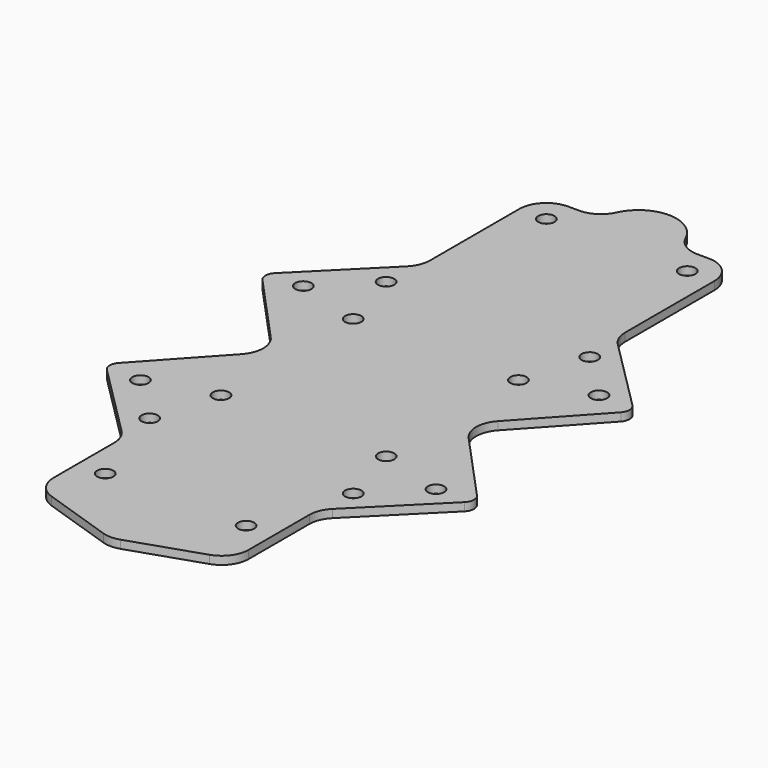
from build123d import *

# Parameters (mm, degrees)
F0_R     = 1.5
F1_DEPTH = 1.5
F2_R     = 5
F3_R     = 2


with BuildPart() as f1:
    # F0 (on Top) → F1 (new body)
    with BuildSketch(Plane.XY):
        with BuildLine():
            Line((34.3576592932, -18), (20.9590200014, -3.3779510381))
            ThreePointArc((20.9590200014, -3.3779510381), (19.6454066855, 0), (20.9590200014, 3.3779510381))
            Line((20.9590200014, 3.3779510381), (34.3576592932, 18))
            Line((34.3576592932, 18), (18, 34.3576592932))
            Line((18, 34.3576592932), (18, 62))
            Line((18, 62), (10.9087121146, 62))
            ThreePointArc((10.9087121146, 62), (8.2084034903, 62.7918729423), (6.3634154002, 64.9166666667))
            ThreePointArc((6.3634154002, 64.9166666667), (0, 69), (-6.3634154002, 64.9166666667))
            ThreePointArc((-6.3634154002, 64.9166666667), (-8.2084034903, 62.7918729423), (-10.9087121146, 62))
            Line((-10.9087121146, 62), (-18, 62))
            Line((-18, 62), (-18, 34.3576592932))
            Line((-18, 34.3576592932), (-34.3576592932, 18))
            Line((-34.3576592932, 18), (-20.9590200014, 3.3779510381))
            ThreePointArc((-20.9590200014, 3.3779510381), (-19.6454066855, 0), (-20.9590200014, -3.3779510381))
            Line((-20.9590200014, -3.3779510381), (-34.3576592932, -18))
            Line((-34.3576592932, -18), (-18, -34.3576592932))
            Line((-18, -34.3576592932), (-18, -54))
            Line((-18, -54), (0, -60))
            Line((0, -60), (18, -54))
            Line((18, -54), (18, -34.3576592932))
            Line((18, -34.3576592932), (34.3576592932, -18))
        make_face()
        with Locations((-13, -44.75)):
            Circle(F0_R, mode=Mode.SUBTRACT)
        with Locations((-27.2708152802, -18.7855339059)):
            Circle(F0_R, mode=Mode.SUBTRACT)
        with Locations((-18.7855339059, -27.2708152802)):
            Circle(F0_R, mode=Mode.SUBTRACT)
        with Locations((-15.25, -15.25)):
            Circle(F0_R, mode=Mode.SUBTRACT)
        with Locations((13, -44.75)):
            Circle(F0_R, mode=Mode.SUBTRACT)
        with Locations((15.25, -15.25)):
            Circle(F0_R, mode=Mode.SUBTRACT)
        with Locations((18.7855339059, -27.2708152802)):
            Circle(F0_R, mode=Mode.SUBTRACT)
        with Locations((27.2708152802, -18.7855339059)):
            Circle(F0_R, mode=Mode.SUBTRACT)
        with Locations((-27.2708152802, 18.7855339059)):
            Circle(F0_R, mode=Mode.SUBTRACT)
        with Locations((-18.7855339059, 27.2708152802)):
            Circle(F0_R, mode=Mode.SUBTRACT)
        with Locations((-15.25, 15.25)):
            Circle(F0_R, mode=Mode.SUBTRACT)
        with Locations((-13, 57)):
            Circle(F0_R, mode=Mode.SUBTRACT)
        with Locations((15.25, 15.25)):
            Circle(F0_R, mode=Mode.SUBTRACT)
        with Locations((27.2708152802, 18.7855339059)):
            Circle(F0_R, mode=Mode.SUBTRACT)
        with Locations((18.7855339059, 27.2708152802)):
            Circle(F0_R, mode=Mode.SUBTRACT)
        with Locations((13, 57)):
            Circle(F0_R, mode=Mode.SUBTRACT)
    extrude(amount=F1_DEPTH)

    # F2
    f2_edges = [f1.edges().sort_by_distance(p)[0] for p in [
        (-18, -54, 0.75),
        (0, -60, 0.75),
        (18, -54, 0.75),
        (-18, 62, 0.75),
        (-18, 34.357659, 0.75),
        (-18, -34.357659, 0.75),
        (18, -34.357659, 0.75),
        (18, 34.357659, 0.75),
        (18, 62, 0.75),
    ]]
    fillet(f2_edges, radius=F2_R)

    # F3
    f3_edges = [f1.edges().sort_by_distance(p)[0] for p in [
        (-34.357659, -18, 0.75),
        (-34.357659, 18, 0.75),
        (34.357659, 18, 0.75),
        (34.357659, -18, 0.75),
    ]]
    fillet(f3_edges, radius=F3_R)


solid = f1.part
